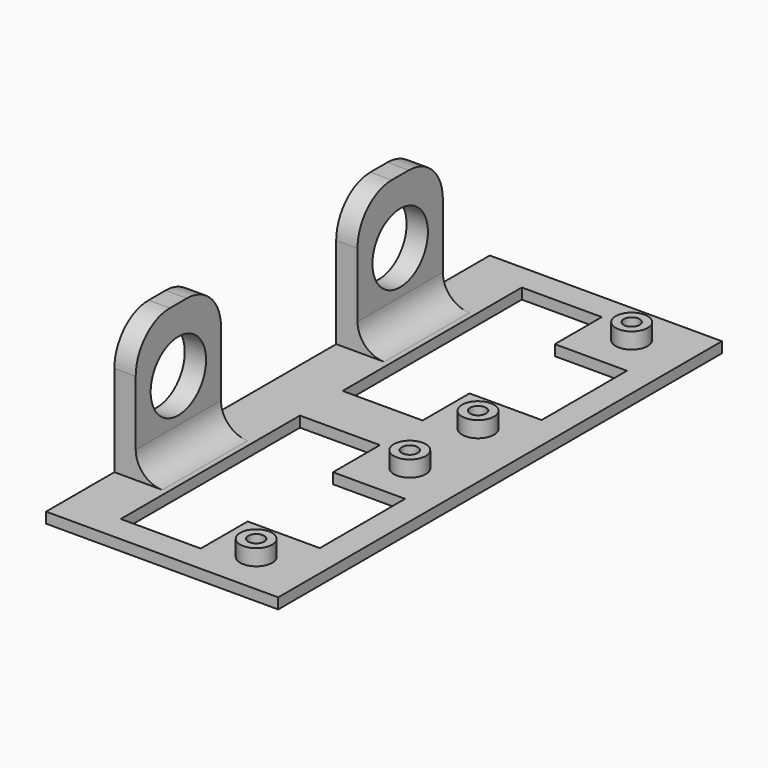
from build123d import *

# Parameters (mm, degrees)
F0_R     = 3
F0_R_2   = 1.5
F1_DEPTH = 2
F0_W     = 43.5258374241
F0_H     = 104
F2_DEPTH = 5
F4_R     = 6.5
F5_DEPTH = 4
F6_R     = 5
F7_R     = 8


# Not quite as in the source:
# - a feature names something its author has since deleted; it is built from what else it names


with BuildPart() as f1:
    # F0 (on Top) → F1 (new body)
    with BuildSketch(Plane.XY):
        Polygon((21, 52), (20, 52), (-20, 52), (-21, 52), (-21, -52), (-20, -52), (20, -52), (21, -52), align=None)
        with Locations((-13, -44)):
            Circle(F0_R, mode=Mode.SUBTRACT)
        with Locations((13, -44)):
            Circle(F0_R, mode=Mode.SUBTRACT)
        with Locations((-13, -8)):
            Circle(F0_R, mode=Mode.SUBTRACT)
        Polygon((-5, -16), (-5, -5), (5, -5), (5, -16), (16, -16), (16, -36), (5, -36), (5, -47), (-5, -47), (-5, -36), (-16, -36), (-16, -16), align=None, mode=Mode.SUBTRACT)
        with Locations((13, -8)):
            Circle(F0_R, mode=Mode.SUBTRACT)
        with Locations((-13, 8)):
            Circle(F0_R, mode=Mode.SUBTRACT)
        with Locations((13, 8)):
            Circle(F0_R, mode=Mode.SUBTRACT)
        with Locations((-13, 44)):
            Circle(F0_R, mode=Mode.SUBTRACT)
        Polygon((-5, 36), (-5, 47), (5, 47), (5, 36), (16, 36), (16, 16), (5, 16), (5, 5), (-5, 5), (-5, 16), (-16, 16), (-16, 36), align=None, mode=Mode.SUBTRACT)
        with Locations((13, 44)):
            Circle(F0_R, mode=Mode.SUBTRACT)
        with Locations((-13, 8)):
            Circle(F0_R)
        with Locations((-13, 8)):
            Circle(F0_R_2, mode=Mode.SUBTRACT)
        with Locations((-13, 44)):
            Circle(F0_R)
        with Locations((-13, 44)):
            Circle(F0_R_2, mode=Mode.SUBTRACT)
    extrude(amount=F1_DEPTH)

    # F0 (on Top) → F2, piece 2 (join)
    with BuildSketch(Plane.XY):
        with Locations((-13, 8)):
            Circle(F0_R)
        with Locations((-13, 8)):
            Circle(F0_R_2, mode=Mode.SUBTRACT)
        with Locations((-13, 44)):
            Circle(F0_R)
        with Locations((-13, 44)):
            Circle(F0_R_2, mode=Mode.SUBTRACT)
        with Locations((13, 44)):
            Circle(F0_R)
        with Locations((13, 44)):
            Circle(F0_R_2, mode=Mode.SUBTRACT)
        with Locations((13, 8)):
            Circle(F0_R)
        with Locations((13, 8)):
            Circle(F0_R_2, mode=Mode.SUBTRACT)
        with Locations((-13, -8)):
            Circle(F0_R)
        with Locations((-13, -8)):
            Circle(F0_R_2, mode=Mode.SUBTRACT)
        with Locations((13, -8)):
            Circle(F0_R)
        with Locations((13, -8)):
            Circle(F0_R_2, mode=Mode.SUBTRACT)
        with Locations((-13, -44)):
            Circle(F0_R)
        with Locations((-13, -44)):
            Circle(F0_R_2, mode=Mode.SUBTRACT)
        with Locations((13, -44)):
            Circle(F0_R)
        with Locations((13, -44)):
            Circle(F0_R_2, mode=Mode.SUBTRACT)
    extrude(amount=F2_DEPTH)


with BuildPart() as f1b:
    # F0 (on Top) → F1, piece 2 (new body)
    with BuildSketch(Plane.XY):
        with Locations((-80.2370812879, 0)):
            Rectangle(F0_W, F0_H)
        with Locations((-69, -44)):
            Circle(F0_R, mode=Mode.SUBTRACT)
        Polygon((-77, -47), (-92, -47), (-92, -5), (-77, -5), (-77, -16), (-63.4741625759, -16), (-63.4741625759, -36), (-77, -36), align=None, mode=Mode.SUBTRACT)
        with Locations((-69, -8)):
            Circle(F0_R, mode=Mode.SUBTRACT)
        with Locations((-69, 8)):
            Circle(F0_R, mode=Mode.SUBTRACT)
        Polygon((-92, 47), (-77, 47), (-77, 36), (-63.4741625759, 36), (-63.4741625759, 16), (-77, 16), (-77, 5), (-92, 5), align=None, mode=Mode.SUBTRACT)
        with Locations((-69, 44)):
            Circle(F0_R, mode=Mode.SUBTRACT)
    extrude(amount=F1_DEPTH)

    # F0 (on Top) → F2 (join)
    with BuildSketch(Plane.XY):
        with Locations((-69, 44)):
            Circle(F0_R)
        with Locations((-69, 44)):
            Circle(F0_R_2, mode=Mode.SUBTRACT)
        with Locations((-69, 8)):
            Circle(F0_R)
        with Locations((-69, 8)):
            Circle(F0_R_2, mode=Mode.SUBTRACT)
        with Locations((-69, -8)):
            Circle(F0_R)
        with Locations((-69, -8)):
            Circle(F0_R_2, mode=Mode.SUBTRACT)
        with Locations((-69, -44)):
            Circle(F0_R)
        with Locations((-69, -44)):
            Circle(F0_R_2, mode=Mode.SUBTRACT)
    extrude(amount=F2_DEPTH)

    # F4 (on face) → F5 (join)
    with BuildSketch(Plane(origin=(-102, 0, 0), x_dir=(0, -1, 0), z_dir=(-1, 0, 0))):
        Polygon((-16, 27.1253478074), (-35.9944990628, 27.1253478074), (-35.9944990628, 0), (-16, 0.4690492824), align=None)
        with Locations((-25.9972495314, 15.1253478074)):
            Circle(F4_R, mode=Mode.SUBTRACT)
        Polygon((16, 0.4690492824), (35.9944990628, 0), (35.9944990628, 27.1253478074), (16, 27.1253478074), align=None)
        with Locations((25.9972495314, 15.1253478074)):
            Circle(F4_R, mode=Mode.SUBTRACT)
    extrude(amount=-F5_DEPTH)

    # F6
    f6_edges = [f1b.edges().sort_by_distance(p)[0] for p in [
        (-98, 25.99725, 2),
        (-98, -25.99725, 2),
    ]]
    fillet(f6_edges, radius=F6_R)

    # F7
    f7_edges = [f1b.edges().sort_by_distance(p)[0] for p in [
        (-100, 35.994499, 27.125348),
        (-100, -16, 27.125348),
        (-100, 16, 27.125348),
        (-100, -35.994499, 27.125348),
    ]]
    fillet(f7_edges, radius=F7_R)


solid = f1b.part
